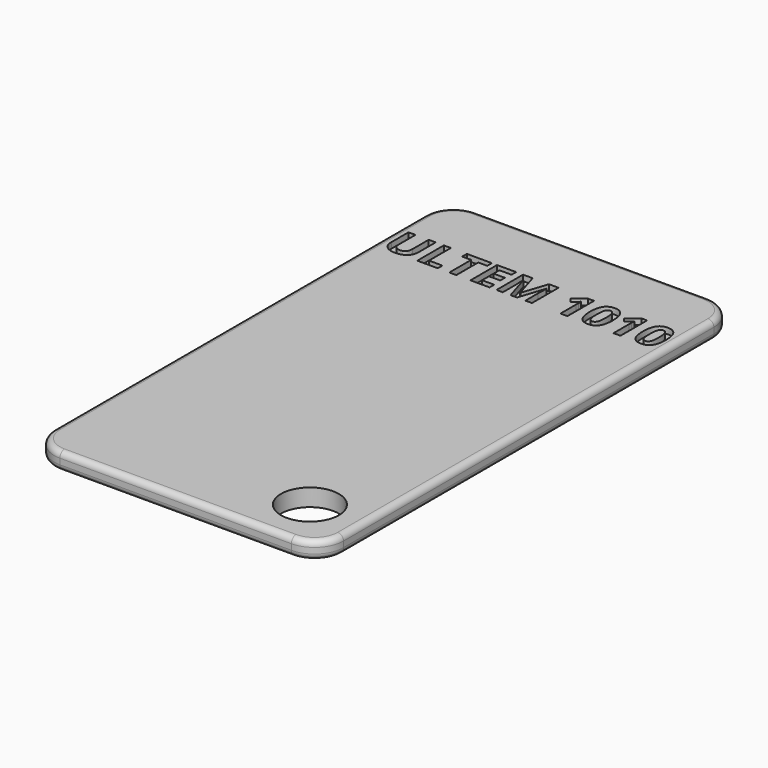
from build123d import *

# Parameters (mm, degrees)
F0_W         = 90
F0_H         = 50
F1_DEPTH     = 3
F2_R         = 1
F3_T1_DEPTH  = 3
F3_T4_ANGLE  = 90
F3_T6_ANGLE  = 90
F3_T8_ANGLE  = 90
F3_T10_ANGLE = 90
F3_T12_ANGLE = 90
F3_T14_ANGLE = 90
F3_T16_ANGLE = 90
F3_T18_ANGLE = 90
F5_ANGLE     = 90
F6_TEXT_SIZE = 8.0334728033
F7_DEPTH     = 1
F8_R         = 5
F9_DEPTH     = 3


# Not quite as in the source:
# - a fillet or chamfer that OpenCascade refuses, or shapes differently, is made with other operations: its cross-section is extruded or revolved along the edge and cut away or added
# - Text() gives the source's letters only with a copy of the font that has no kerning and outlines rounded to 1/6400 em; it was checked with that copy


with BuildPart() as f1:
    # F0 (on Top) → F1 (new body)
    with BuildSketch(Plane.XY):
        Rectangle(F0_W, F0_H)
    extrude(amount=F1_DEPTH)

    # F2
    f2_edges = [f1.edges().sort_by_distance(p)[0] for p in [
        (0, 25, 3),
        (-45, 0, 3),
        (0, -25, 3),
        (45, 0, 3),
        (0, 25, 0),
        (-45, 0, 0),
        (0, -25, 0),
        (45, 0, 0),
    ]]
    fillet(f2_edges, radius=F2_R)

    # F3: fillet of radius 5 on 4 edges, made by hand

    # F3_s2 → F3_t1 (cut)
    with BuildSketch(Plane.XY):
        with BuildLine():
            ThreePointArc((45, -20), (43.5355339059, -23.5355339059), (40, -25))
            Line((40, -25), (45, -25))
            Line((45, -25), (45, -20))
        make_face()
        with BuildLine():
            ThreePointArc((40, 25), (43.5355339059, 23.5355339059), (45, 20))
            Line((45, 20), (45, 25))
            Line((45, 25), (40, 25))
        make_face()
        with BuildLine():
            ThreePointArc((-40, 25), (-43.5355339059, 23.5355339059), (-45, 20))
            Line((-45, 20), (-45, 25))
            Line((-45, 25), (-40, 25))
        make_face()
        with BuildLine():
            ThreePointArc((-45, -20), (-43.5355339059, -23.5355339059), (-40, -25))
            Line((-40, -25), (-45, -25))
            Line((-45, -25), (-45, -20))
        make_face()
    extrude(amount=F3_T1_DEPTH, mode=Mode.SUBTRACT)

    # F3_s3 → F3_t4 (revolve, cut)
    with BuildSketch(Plane.YZ.offset(-40)):
        with BuildLine():
            ThreePointArc((-24, 0), (-24.7071067812, 0.2928932188), (-25, 1))
            Line((-25, 1), (-25, 0))
            Line((-25, 0), (-24, 0))
        make_face()
    revolve(axis=Axis((-40, -20, 0), (0, 0, -1)), revolution_arc=F3_T4_ANGLE, mode=Mode.SUBTRACT)

    # F3_s5 → F3_t6 (revolve, cut)
    with BuildSketch(Plane.XZ.offset(20)):
        with BuildLine():
            ThreePointArc((-44, 3), (-44.7071067812, 2.7071067812), (-45, 2))
            Line((-45, 2), (-45, 3))
            Line((-45, 3), (-44, 3))
        make_face()
    revolve(axis=Axis((-40, -20, 3), (0, 0, 1)), revolution_arc=F3_T6_ANGLE, mode=Mode.SUBTRACT)

    # F3_s7 → F3_t8 (revolve, cut)
    with BuildSketch(Plane.XZ.offset(-20)):
        with BuildLine():
            ThreePointArc((-44, 0), (-44.7071067812, 0.2928932188), (-45, 1))
            Line((-45, 1), (-45, 0))
            Line((-45, 0), (-44, 0))
        make_face()
    revolve(axis=Axis((-40, 20, 0), (0, 0, -1)), revolution_arc=F3_T8_ANGLE, mode=Mode.SUBTRACT)

    # F3_s9 → F3_t10 (revolve, cut)
    with BuildSketch(Plane.YZ.offset(-40)):
        with BuildLine():
            ThreePointArc((24, 3), (24.7071067812, 2.7071067812), (25, 2))
            Line((25, 2), (25, 3))
            Line((25, 3), (24, 3))
        make_face()
    revolve(axis=Axis((-40, 20, 3), (0, 0, 1)), revolution_arc=F3_T10_ANGLE, mode=Mode.SUBTRACT)

    # F3_s11 → F3_t12 (revolve, cut)
    with BuildSketch(Plane.YZ.offset(40)):
        with BuildLine():
            ThreePointArc((24, 0), (24.7071067812, 0.2928932188), (25, 1))
            Line((25, 1), (25, 0))
            Line((25, 0), (24, 0))
        make_face()
    revolve(axis=Axis((40, 20, 0), (0, 0, -1)), revolution_arc=F3_T12_ANGLE, mode=Mode.SUBTRACT)

    # F3_s13 → F3_t14 (revolve, cut)
    with BuildSketch(Plane.XZ.offset(-20)):
        with BuildLine():
            ThreePointArc((44, 3), (44.7071067812, 2.7071067812), (45, 2))
            Line((45, 2), (45, 3))
            Line((45, 3), (44, 3))
        make_face()
    revolve(axis=Axis((40, 20, 3), (0, 0, 1)), revolution_arc=F3_T14_ANGLE, mode=Mode.SUBTRACT)

    # F3_s15 → F3_t16 (revolve, cut)
    with BuildSketch(Plane.XZ.offset(20)):
        with BuildLine():
            ThreePointArc((44, 0), (44.7071067812, 0.2928932188), (45, 1))
            Line((45, 1), (45, 0))
            Line((45, 0), (44, 0))
        make_face()
    revolve(axis=Axis((40, -20, 0), (0, 0, -1)), revolution_arc=F3_T16_ANGLE, mode=Mode.SUBTRACT)

    # F3_s17 → F3_t18 (revolve, cut)
    with BuildSketch(Plane.YZ.offset(40)):
        with BuildLine():
            ThreePointArc((-24, 3), (-24.7071067812, 2.7071067812), (-25, 2))
            Line((-25, 2), (-25, 3))
            Line((-25, 3), (-24, 3))
        make_face()
    revolve(axis=Axis((40, -20, 3), (0, 0, 1)), revolution_arc=F3_T18_ANGLE, mode=Mode.SUBTRACT)


with BuildPart() as f1_1:
    # F5: moved
    add(f1.part.rotate(Axis((0, 0, 16.4477843791), (0, 0, 1)), F5_ANGLE))

    # F6 (on face) → F7 (cut)
    with BuildSketch(Plane.XY.offset(3)):
        with Locations((-24, 28.6952870173)):
            Text('ULTEM 1010', F6_TEXT_SIZE, font='Open Sans', font_style=FontStyle.BOLD, text_align=(TextAlign.LEFT, TextAlign.BOTTOM))
    extrude(amount=-F7_DEPTH, mode=Mode.SUBTRACT)

    # F8 (on face) → F9 (cut)
    with BuildSketch(Plane.XY.offset(3)):
        with Locations((16, -36)):
            Circle(F8_R)
    extrude(amount=-F9_DEPTH, mode=Mode.SUBTRACT)


solid = f1_1.part
